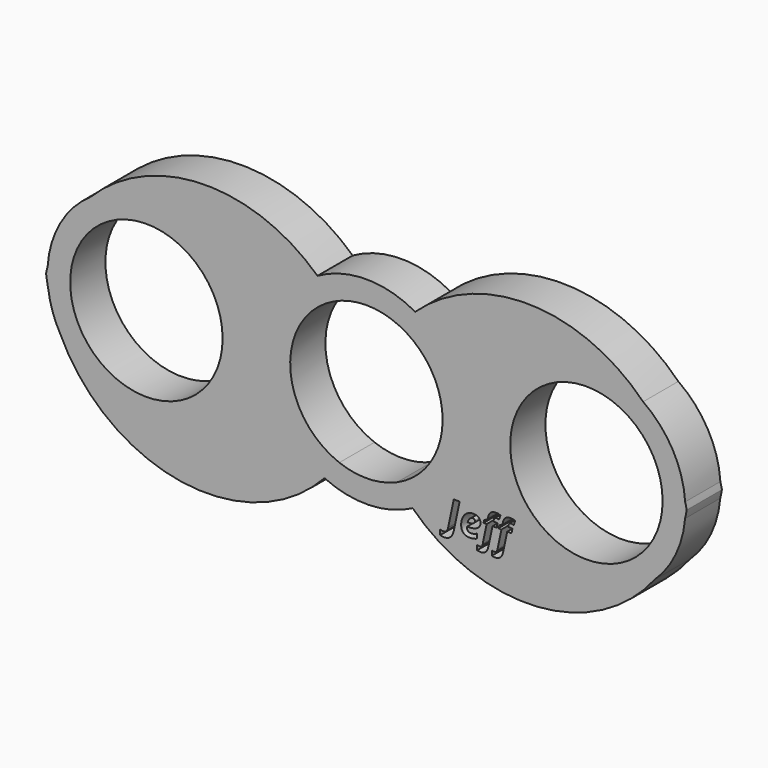
from build123d import *

# Parameters (mm, degrees)
F2_R         = 10.9982
F3_DEPTH     = 6.35
F4_TEXT_SIZE = 5.698718855
F5_DEPTH     = 6.351


# Not quite as in the source:
# - Text() gives the source's letters only with a copy of the font that has no kerning and outlines rounded to 1/6400 em; it was checked with that copy


with BuildPart() as f3:
    # F2 (on Front) → F3 (new body)
    with BuildSketch(Plane.XZ):
        with BuildLine():
            ThreePointArc((-44.1863266757, -7.0335222376), (-28.113474263, -13.8169583054), (-17.4625, 0))
            ThreePointArc((-17.4625, 0), (-25.093279917, 12.6420225434), (-39.8346062448, 11.7801442315))
            ThreePointArc((-39.8346062448, 11.7801442315), (-43.64773478, 6.7776467648), (-46.0061181686, 0.9464412356))
            ThreePointArc((-46.0061181686, 0.9464412356), (-46.0296767311, -0.4727459191), (-45.9123048268, -1.8872674007))
            ThreePointArc((-45.9123048268, -1.8872674007), (-45.1997207675, -4.5108384486), (-44.1863266757, -7.0335222376))
        make_face()
        with Locations((-31.75, 0)):
            Circle(F2_R, mode=Mode.SUBTRACT)
        with BuildLine():
            ThreePointArc((-39.8346062448, 11.7801442315), (-25.093279917, 12.6420225434), (-17.4625, 0))
            ThreePointArc((-17.4625, 0), (-28.113474263, -13.8169583054), (-44.1863266757, -7.0335222376))
            ThreePointArc((-44.1863266757, -7.0335222376), (-26.6834466249, -20.1232804847), (-6.0383744332, -12.948771774))
            ThreePointArc((-6.0383744332, -12.948771774), (-14.2759396663, -0.5746328345), (-7.0595767645, 12.4215551424))
            ThreePointArc((-7.0595767645, 12.4215551424), (-23.5763872183, 18.7076453518), (-39.8346062448, 11.7801442315))
        make_face()
        with BuildLine():
            ThreePointArc((-46.0061181686, 0.9464412356), (-43.64773478, 6.7776467648), (-39.8346062448, 11.7801442315))
            ThreePointArc((-39.8346062448, 11.7801442315), (-44.1644783209, 7.0720141593), (-46.0061181686, 0.9464412356))
        make_face()
        with BuildLine():
            ThreePointArc((-45.9123048268, -1.8872674007), (-45.2959508401, -4.543112599), (-44.1863266757, -7.0335222376))
            ThreePointArc((-44.1863266757, -7.0335222376), (-45.1997207675, -4.5108384486), (-45.9123048268, -1.8872674007))
        make_face()
        with BuildLine():
            ThreePointArc((-45.9123048268, -1.8872674007), (-46.0296767311, -0.4727459191), (-46.0061181686, 0.9464412356))
            ThreePointArc((-46.0061181686, 0.9464412356), (-46.121926134, 0.4743616394), (-46.228, 0))
            ThreePointArc((-46.228, 0), (-46.089538692, -0.946876566), (-45.9123048268, -1.8872674007))
        make_face()
        with BuildLine():
            ThreePointArc((7.037012799, 12.4343518977), (-0.0129700567, 14.287494113), (-7.0595767645, 12.4215551424))
            ThreePointArc((-7.0595767645, 12.4215551424), (-5.8497132573, 11.2174536913), (-4.7299221239, 9.9291610895))
            ThreePointArc((-4.7299221239, 9.9291610895), (-0.010160638, 10.9981953066), (4.7115680355, 9.9378835718))
            ThreePointArc((4.7115680355, 9.9378835718), (5.8291605439, 11.2281559319), (7.037012799, 12.4343518977))
        make_face()
        with BuildLine():
            ThreePointArc((-4.7299221239, 9.9291610895), (-5.8497132573, 11.2174536913), (-7.0595767645, 12.4215551424))
            ThreePointArc((-7.0595767645, 12.4215551424), (-14.2759396663, -0.5746328345), (-6.0383744332, -12.948771774))
            ThreePointArc((-6.0383744332, -12.948771774), (-4.9227302487, -11.6543432485), (-3.9049809544, -10.2816111085))
            ThreePointArc((-3.9049809544, -10.2816111085), (-10.9890498226, -0.448539003), (-4.7299221239, 9.9291610895))
        make_face()
        with BuildLine():
            ThreePointArc((-3.9049809544, -10.2816111085), (-4.9227302487, -11.6543432485), (-6.0383744332, -12.948771774))
            ThreePointArc((-6.0383744332, -12.948771774), (0.3536815145, -14.2831217049), (6.6718610916, -12.6340383815))
            ThreePointArc((6.6718610916, -12.6340383815), (5.4970075205, -11.3945711128), (4.4153548205, -10.0729859053))
            ThreePointArc((4.4153548205, -10.0729859053), (0.2756836768, -10.9947442785), (-3.9049809544, -10.2816111085))
        make_face()
        with BuildLine():
            ThreePointArc((39.9398856102, 11.7071956481), (23.6359207408, 18.7436686303), (7.037012799, 12.4343518977))
            ThreePointArc((7.037012799, 12.4343518977), (12.34248712, 7.1969207264), (14.2875, 0))
            ThreePointArc((14.2875, 0), (12.2363571294, -7.3759216679), (6.6718610916, -12.6340383815))
            ThreePointArc((6.6718610916, -12.6340383815), (24.6452730711, -19.3021441211), (41.5978965979, -10.3514051629))
            ThreePointArc((41.5978965979, -10.3514051629), (17.5026892298, -1.0708837793), (39.9398856102, 11.7071956481))
        make_face()
        with BuildLine():
            ThreePointArc((14.2875, 0), (12.34248712, 7.1969207264), (7.037012799, 12.4343518977))
            ThreePointArc((7.037012799, 12.4343518977), (5.8291605439, 11.2281559319), (4.7115680355, 9.9378835718))
            ThreePointArc((4.7115680355, 9.9378835718), (9.294599798, 5.8796953863), (10.9982, 0))
            ThreePointArc((10.9982, 0), (9.2065563222, -6.0166206401), (4.4153548205, -10.0729859053))
            ThreePointArc((4.4153548205, -10.0729859053), (5.4970075205, -11.3945711128), (6.6718610916, -12.6340383815))
            ThreePointArc((6.6718610916, -12.6340383815), (12.2363571294, -7.3759216679), (14.2875, 0))
        make_face()
        with BuildLine():
            ThreePointArc((46.0054268898, 0.9567969682), (44.1935035762, 7.0208172601), (39.9398856102, 11.7071956481))
            ThreePointArc((39.9398856102, 11.7071956481), (43.6872592459, 6.7351863757), (46.0054268898, 0.9567969682))
        make_face()
        with BuildLine():
            ThreePointArc((46.0054268898, 0.9567969682), (43.6872592459, 6.7351863757), (39.9398856102, 11.7071956481))
            ThreePointArc((39.9398856102, 11.7071956481), (17.5026892298, -1.0708837793), (41.5978965979, -10.3514051629))
            ThreePointArc((41.5978965979, -10.3514051629), (44.2984126843, -5.9974118306), (45.9902247178, -1.1613165963))
            ThreePointArc((45.9902247178, -1.1613165963), (46.0256762871, -0.5811392237), (46.0375, 0))
            ThreePointArc((46.0375, 0), (46.0294794712, 0.478667192), (46.0054268898, 0.9567969682))
        make_face()
        with Locations((31.75, 0)):
            Circle(F2_R, mode=Mode.SUBTRACT)
        with BuildLine():
            ThreePointArc((45.9902247178, -1.1613165963), (44.2984126843, -5.9974118306), (41.5978965979, -10.3514051629))
            ThreePointArc((41.5978965979, -10.3514051629), (44.6408428388, -6.1610735391), (45.9902247178, -1.1613165963))
        make_face()
        with BuildLine():
            ThreePointArc((46.228, 0), (46.1216876487, 0.4795555989), (46.0054268898, 0.9567969682))
            ThreePointArc((46.0054268898, 0.9567969682), (46.0294794712, 0.478667192), (46.0375, 0))
            ThreePointArc((46.0375, 0), (46.0256762871, -0.5811392237), (45.9902247178, -1.1613165963))
            ThreePointArc((45.9902247178, -1.1613165963), (46.116442402, -0.5821590974), (46.228, 0))
        make_face()
    extrude(amount=F3_DEPTH)

    # F4 (on Front) → F5 (cut, through all)
    with BuildSketch(Plane.XZ):
        with Locations((11.5399090573, -13.6484313084)):
            Text('Jeff', F4_TEXT_SIZE, font='Open Sans', font_style=FontStyle.BOLDITALIC, text_align=(TextAlign.LEFT, TextAlign.BOTTOM))
    extrude(amount=F5_DEPTH, mode=Mode.SUBTRACT)


solid = f3.part
